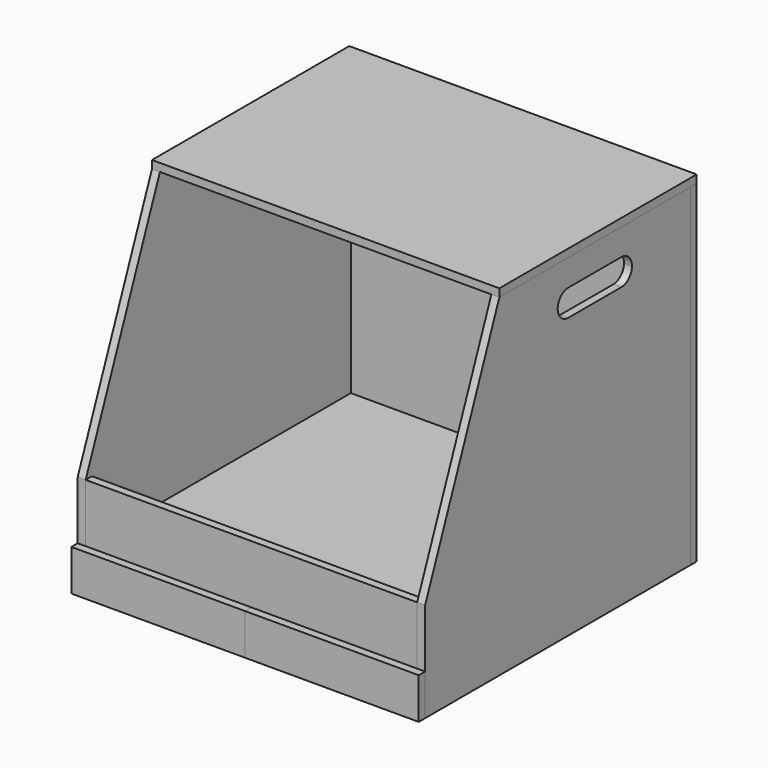
from build123d import *

# Parameters (mm, degrees)
F0_W      = 500
F0_H      = 500
F1_DEPTH  = 12
F2_W      = 500
F2_H      = 50
F3_DEPTH  = 6
F6_DEPTH  = 6
F14_DEPTH = 6
F15_R     = 19.99999
F19_DEPTH = 6
F22_DEPTH = 12
F25_DEPTH = 6
F27_W     = 12
F27_H     = 320
F28_DEPTH = 44
F31_W     = 196
F31_H     = 12
F32_DEPTH = 44
F37_DEPTH = 3
F43_DEPTH = 12


# Not quite as in the source:
# - a fillet or chamfer is up to 0.001 mm smaller than in the source, because OpenCascade refuses the exact size


with BuildPart() as f1:
    # F0 (on Top) → F1 (new body)
    with BuildSketch(Plane.XY):
        Rectangle(F0_W, F0_H)
    extrude(amount=F1_DEPTH)


with BuildPart() as f3:
    # F2 (on Right) → F3 (new body, symmetric)
    with BuildSketch(Plane.YZ):
        Rectangle(F2_W, F2_H)
    extrude(amount=F3_DEPTH, both=True)


with BuildPart() as f3_1:
    # F4: moved
    add(f3.part.moved(Location((0, 0, -25))))


with BuildPart() as f6:
    # F5 (on Front) → F6 (new body, symmetric)
    with BuildSketch(Plane.XZ):
        Polygon((-250, -25), (250, -25), (250, 25), (6, 25), (6, 0), (-6, 0), (-6, 25), (-250, 25), align=None)
    extrude(amount=F6_DEPTH, both=True)


with BuildPart() as f6_1:
    # F7: moved
    add(f6.part.moved(Location((0, 80, -25))))


with BuildPart() as f8_1:
    # F8: copy of F6
    add(f6_1.part)


with BuildPart() as f3_2:
    add(f3_1.part)

    # F10: cut F6
    add(f6_1.part, mode=Mode.SUBTRACT)


with BuildPart() as f11_1:
    # F11: copy of F6
    add(f6_1.part.moved(Location((0, 164, 0))))


with BuildPart() as f3_3:
    add(f3_2.part)

    # F12: cut F11_1
    add(f11_1.part, mode=Mode.SUBTRACT)


with BuildPart() as f14:
    # F13 (on Right) → F14 (new body, symmetric)
    with BuildSketch(Plane.YZ):
        Polygon((250, -50), (250, 0), (250, 452), (70, 452), (-110, 452), (-250, 100), (-250, -50), align=None)
        Polygon((0, 412), (70, 412), (140, 412), (140, 372), (0, 372), align=None, mode=Mode.SUBTRACT)
    extrude(amount=F14_DEPTH, both=True)

    # F15 (radius 20 in the source; OpenCascade refuses exactly that, so slightly less here)
    f15_edges = [f14.edges().sort_by_distance(p)[0] for p in [
        (0, 140, 372),
        (0, 140, 412),
        (0, 0, 412),
        (0, 0, 372),
    ]]
    fillet(f15_edges, radius=F15_R)


with BuildPart() as f14_1:
    # F16: moved
    add(f14.part.moved(Location((-256, 0, 0))))


with BuildPart() as f17_1:
    # F17: copy of F14
    add(f14_1.part.moved(Location((512, 0, 0))))


with BuildPart() as f19:
    # F18 (on Front) → F19 (new body, symmetric)
    with BuildSketch(Plane.XZ):
        Polygon((-262, 452), (-262, 0), (-262, -50), (262, -50), (262, 452), align=None)
    extrude(amount=F19_DEPTH, both=True)


with BuildPart() as f19_1:
    # F20: moved
    add(f19.part.moved(Location((0, 256, 0))))


with BuildPart() as f22:
    # F21 (on face) → F22 (new body)
    with BuildSketch(Plane.XY.offset(12)):
        Polygon((262, 262), (0, 262), (-262, 262), (-262, -110), (262, -110), align=None)
    extrude(amount=F22_DEPTH)


with BuildPart() as f22_1:
    # F23: moved
    add(f22.part.moved(Location((0, 0, 440))))


with BuildPart() as f25:
    # F24 (on Front) → F25 (new body, symmetric)
    with BuildSketch(Plane.XZ):
        Polygon((-250, 12), (0, 12), (250, 12), (250, 100), (-250, 100), align=None)
    extrude(amount=F25_DEPTH, both=True)


with BuildPart() as f25_1:
    # F26: moved
    add(f25.part.moved(Location((0, -244, 0))))


with BuildPart() as f28:
    # F27 (on Top) → F28 (new body)
    with BuildSketch(Plane.XY):
        with Locations((-24, -90)):
            Rectangle(F27_W, F27_H)
    extrude(amount=F28_DEPTH)


with BuildPart() as f28_1:
    # F29: moved
    add(f28.part.moved(Location((0, 0, -48))))


with BuildPart() as f30_1:
    # F30: copy of F28
    add(f28_1.part.moved(Location((-208, 0, 0))))


with BuildPart() as f32:
    # F31 (on Top) → F32 (new body)
    with BuildSketch(Plane.XY):
        with Locations((-128, -244)):
            Rectangle(F31_W, F31_H)
    extrude(amount=-F32_DEPTH)


with BuildPart() as f32_1:
    # F33: moved
    add(f32.part.moved(Location((0, 0, -4))))


with BuildPart() as f34_1:
    # F34: copy of F32
    add(f32_1.part.moved(Location((0, 308, 0))))


with BuildPart() as f35_1:
    # F35: copy of F32
    add(f32_1.part.moved(Location((256, 0, 0))))


with BuildPart() as f35_2:
    # F35: copy of F30_1
    add(f30_1.part.moved(Location((256, 0, 0))))


with BuildPart() as f35_3:
    # F35: copy of F28
    add(f28_1.part.moved(Location((256, 0, 0))))


with BuildPart() as f35_4:
    # F35: copy of F34_1
    add(f34_1.part.moved(Location((256, 0, 0))))


with BuildPart() as f37:
    # F36 (on Top) → F37 (new body)
    with BuildSketch(Plane.XY):
        Polygon((-24, -244), (-24, 0), (-24, 64), (-232, 64), (-232, -244), align=None)
    extrude(amount=F37_DEPTH)


with BuildPart() as f37_1:
    # F38: moved
    add(f37.part.moved(Location((0, 0, -44))))


with BuildPart() as f39_1:
    # F39: copy of F37
    add(f37_1.part.moved(Location((256, 0, 0))))


with BuildPart() as f30_1_1:
    add(f30_1.part)

    # F40: cut F37
    add(f37_1.part, mode=Mode.SUBTRACT)


with BuildPart() as f32_2:
    add(f32_1.part)

    # F40: cut F37
    add(f37_1.part, mode=Mode.SUBTRACT)


with BuildPart() as f28_2:
    add(f28_1.part)

    # F40: cut F37
    add(f37_1.part, mode=Mode.SUBTRACT)


with BuildPart() as f34_1_1:
    add(f34_1.part)

    # F40: cut F37
    add(f37_1.part, mode=Mode.SUBTRACT)


with BuildPart() as f35_1_1:
    add(f35_1.part)

    # F41: cut F39_1
    add(f39_1.part, mode=Mode.SUBTRACT)


with BuildPart() as f35_3_1:
    add(f35_3.part)

    # F41: cut F39_1
    add(f39_1.part, mode=Mode.SUBTRACT)


with BuildPart() as f35_4_1:
    add(f35_4.part)

    # F41: cut F39_1
    add(f39_1.part, mode=Mode.SUBTRACT)


with BuildPart() as f35_2_1:
    add(f35_2.part)

    # F41: cut F39_1
    add(f39_1.part, mode=Mode.SUBTRACT)


with BuildPart() as f43:
    # F42 (on Front) → F43 (new body)
    with BuildSketch(Plane.XZ):
        Polygon((0, 12), (0, 0), (0, -50), (262, -50), (262, 12), align=None)
    extrude(amount=F43_DEPTH)


with BuildPart() as f43_1:
    # F44: moved
    add(f43.part.moved(Location((0, -250, 0))))


with BuildPart() as f45_1:
    # F45: copy of F43
    add(f43_1.part.moved(Location((-262, 0, 0))))


solid = Compound([f1.part, f6_1.part, f11_1.part, f3_3.part, f14_1.part, f17_1.part, f19_1.part, f22_1.part, f25_1.part, f37_1.part, f39_1.part, f30_1_1.part, f32_2.part, f28_2.part, f34_1_1.part, f35_1_1.part, f35_3_1.part, f35_4_1.part, f35_2_1.part, f43_1.part, f45_1.part])
